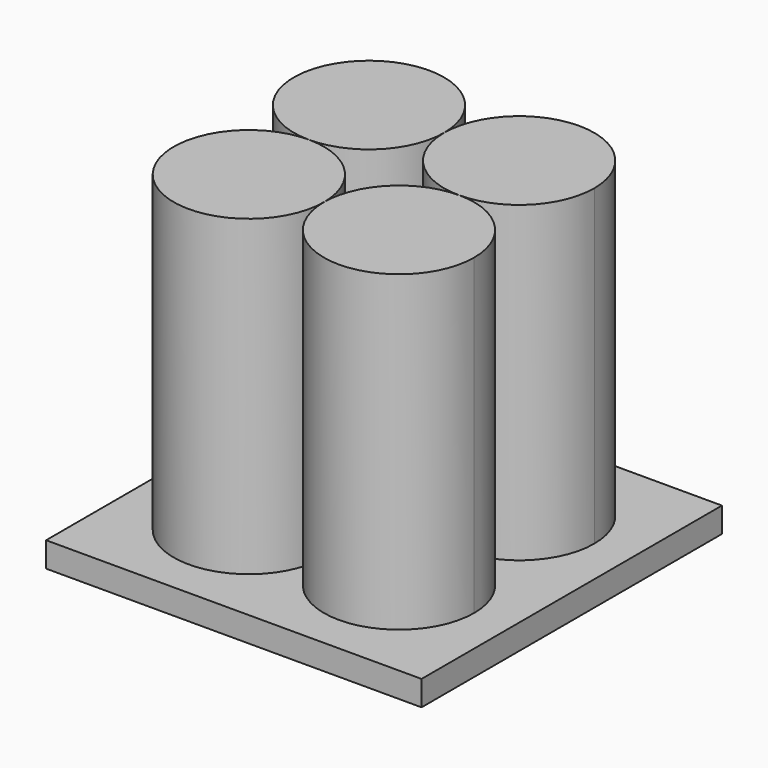
from build123d import *

# Parameters (mm, degrees)
F1_DEPTH = 63.5
F2_W     = 76.2
F2_H     = 5.08
F3_DEPTH = 38.1


# Not quite as in the source:
# - a feature names something its author has since deleted; it is built from what else it names


with BuildPart() as f1:
    # F0 (on Top) → F1 (new body)
    with BuildSketch(Plane.XY):
        with BuildLine():
            ThreePointArc((-15.2400000598, 0), (-26.0163073241, -26.0163073664), (0, -15.24))
            ThreePointArc((0, -15.24), (-4.4636926759, -4.4636926336), (-15.2400000598, 0))
        make_face()
    extrude(amount=F1_DEPTH)


with BuildPart() as f1b:
    # F0 (on Top) → F1, piece 2 (new body)
    with BuildSketch(Plane.XY):
        with BuildLine():
            ThreePointArc((15.24, 0), (4.4636926547, -4.4636926547), (0, -15.24))
            ThreePointArc((0, -15.24), (15.24, -30.48), (30.48, -15.24))
            ThreePointArc((30.48, -15.24), (26.0163073453, -4.4636926547), (15.24, 0))
        make_face()
    extrude(amount=F1_DEPTH)


with BuildPart() as f1c:
    # F0 (on Top) → F1, piece 3 (new body)
    with BuildSketch(Plane.XY):
        with BuildLine():
            ThreePointArc((0, 15.24), (-26.0163073241, 26.0163073664), (-15.2400000598, 0))
            ThreePointArc((-15.2400000598, 0), (-4.4636926759, 4.4636926336), (0, 15.24))
        make_face()
    extrude(amount=F1_DEPTH)


with BuildPart() as f1d:
    # F0 (on Top) → F1, piece 4 (new body)
    with BuildSketch(Plane.XY):
        with BuildLine():
            ThreePointArc((0, 15.24), (4.4636926547, 4.4636926547), (15.24, 0))
            ThreePointArc((15.24, 0), (26.0163073453, 4.4636926547), (30.48, 15.24))
            ThreePointArc((30.48, 15.24), (15.24, 30.48), (0, 15.24))
        make_face()
    extrude(amount=F1_DEPTH)


with BuildPart() as f3:
    # F2 (on Front) → F3 (new body, symmetric)
    with BuildSketch(Plane.XZ):
        with Locations((0, -2.54)):
            Rectangle(F2_W, F2_H)
    extrude(amount=F3_DEPTH, both=True)


solid = Compound([f1.part, f1b.part, f1c.part, f1d.part, f3.part])
